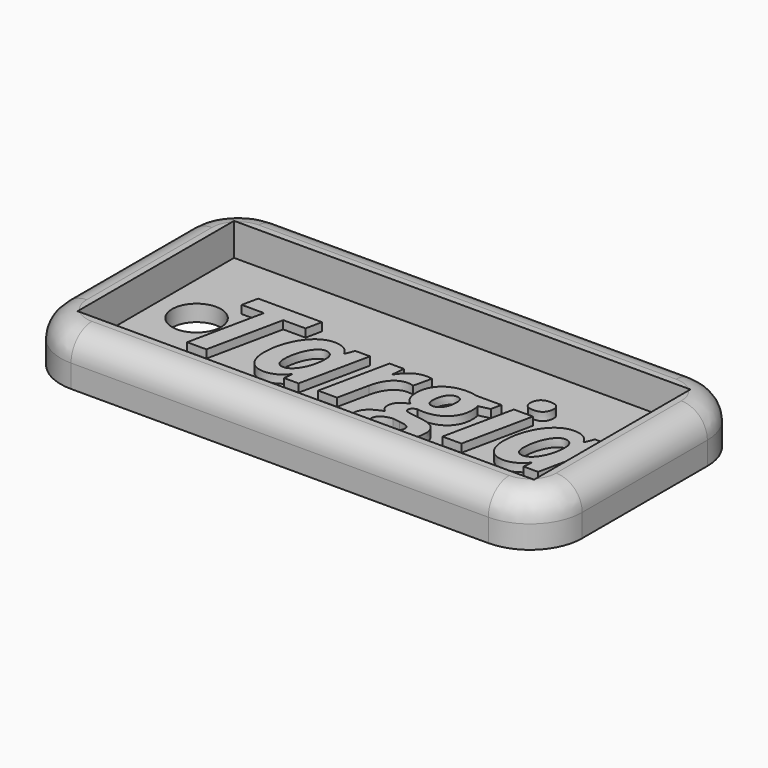
from build123d import *

# Parameters (mm, degrees)
F0_W         = 44.45
F0_H         = 19.05
F0_R         = 2.38125
F1_DEPTH     = 1.5875
F0_W_2       = 50.8
F0_H_2       = 25.4
F2_DEPTH     = 4.7625
F3_R         = 5.08
F4_T1_DEPTH  = 40.64
F4_T3_DEPTH  = 15.24
F4_T6_ANGLE  = 90
F4_T8_ANGLE  = 90
F4_T10_ANGLE = 90
F4_T12_ANGLE = 90
F5_TEXT_SIZE = 12.5911391098
F6_DEPTH     = 0.79375


# Not quite as in the source:
# - a fillet or chamfer that OpenCascade refuses, or shapes differently, is made with other operations: its cross-section is extruded or revolved along the edge and cut away or added
# - Text() gives the source's letters only with a copy of the font that has no kerning and outlines rounded to 1/6400 em; it was checked with that copy


with BuildPart() as f1:
    # F0 (on Top) → F1 (new body)
    with BuildSketch(Plane.XY):
        with Locations((25.4, 12.7)):
            Rectangle(F0_W, F0_H)
        with Locations((7.14375, 12.7)):
            Circle(F0_R, mode=Mode.SUBTRACT)
    extrude(amount=F1_DEPTH)

    # F0 (on Top) → F2 (join)
    with BuildSketch(Plane.XY):
        with Locations((25.4, 12.7)):
            Rectangle(F0_W_2, F0_H_2)
        with Locations((25.4, 12.7)):
            Rectangle(F0_W, F0_H, mode=Mode.SUBTRACT)
    extrude(amount=F2_DEPTH)

    # F3
    f3_edges = [f1.edges().sort_by_distance(p)[0] for p in [
        (50.8, 0, 2.38125),
        (0, 0, 2.38125),
        (50.8, 25.4, 2.38125),
        (0, 25.4, 2.38125),
    ]]
    fillet(f3_edges, radius=F3_R)

    # F4: fillet of radius 2.54 on 8 edges, made by hand

    # F4_s2 → F4_t1 (cut)
    with BuildSketch(Plane.YZ.offset(5.08)):
        with BuildLine():
            ThreePointArc((0, 2.2225), (0.7439487758, 4.0185512242), (2.54, 4.7625))
            Line((2.54, 4.7625), (0, 4.7625))
            Line((0, 4.7625), (0, 2.2225))
        make_face()
        with BuildLine():
            ThreePointArc((25.4, 2.2225), (24.6560512242, 4.0185512242), (22.86, 4.7625))
            Line((22.86, 4.7625), (25.4, 4.7625))
            Line((25.4, 4.7625), (25.4, 2.2225))
        make_face()
    extrude(amount=F4_T1_DEPTH, mode=Mode.SUBTRACT)

    # F4_s4 → F4_t3 (cut)
    with BuildSketch(Plane.XZ.offset(-20.32)):
        with BuildLine():
            ThreePointArc((0, 2.2225), (0.7439487758, 4.0185512242), (2.54, 4.7625))
            Line((2.54, 4.7625), (0, 4.7625))
            Line((0, 4.7625), (0, 2.2225))
        make_face()
        with BuildLine():
            ThreePointArc((50.8, 2.2225), (50.0560512242, 4.0185512242), (48.26, 4.7625))
            Line((48.26, 4.7625), (50.8, 4.7625))
            Line((50.8, 4.7625), (50.8, 2.2225))
        make_face()
    extrude(amount=F4_T3_DEPTH, mode=Mode.SUBTRACT)

    # F4_s5 → F4_t6 (revolve, cut)
    with BuildSketch(Plane.XZ.offset(-20.32)):
        with BuildLine():
            ThreePointArc((0, 2.2225), (0.7439487758, 4.0185512242), (2.54, 4.7625))
            Line((2.54, 4.7625), (0, 4.7625))
            Line((0, 4.7625), (0, 2.2225))
        make_face()
    revolve(axis=Axis((5.08, 20.32, 4.7625), (0, 0, -1)), revolution_arc=F4_T6_ANGLE, mode=Mode.SUBTRACT)

    # F4_s7 → F4_t8 (revolve, cut)
    with BuildSketch(Plane.XZ.offset(-5.08)):
        with BuildLine():
            ThreePointArc((0, 2.2225), (0.7439487758, 4.0185512242), (2.54, 4.7625))
            Line((2.54, 4.7625), (0, 4.7625))
            Line((0, 4.7625), (0, 2.2225))
        make_face()
    revolve(axis=Axis((5.08, 5.08, 4.7625), (0, 0, 1)), revolution_arc=F4_T8_ANGLE, mode=Mode.SUBTRACT)

    # F4_s9 → F4_t10 (revolve, cut)
    with BuildSketch(Plane.XZ.offset(-20.32)):
        with BuildLine():
            ThreePointArc((50.8, 2.2225), (50.0560512242, 4.0185512242), (48.26, 4.7625))
            Line((48.26, 4.7625), (50.8, 4.7625))
            Line((50.8, 4.7625), (50.8, 2.2225))
        make_face()
    revolve(axis=Axis((45.72, 20.32, 4.7625), (0, 0, 1)), revolution_arc=F4_T10_ANGLE, mode=Mode.SUBTRACT)

    # F4_s11 → F4_t12 (revolve, cut)
    with BuildSketch(Plane.YZ.offset(45.72)):
        with BuildLine():
            ThreePointArc((0, 2.2225), (0.7439487758, 4.0185512242), (2.54, 4.7625))
            Line((2.54, 4.7625), (0, 4.7625))
            Line((0, 4.7625), (0, 2.2225))
        make_face()
    revolve(axis=Axis((45.72, 5.08, 4.7625), (0, 0, 1)), revolution_arc=F4_T12_ANGLE, mode=Mode.SUBTRACT)

    # F5 (on face) → F6 (join)
    with BuildSketch(Plane.XY.offset(1.5875)):
        with Locations((8.3821003724, 7.9563454469)):
            Text('Targia', F5_TEXT_SIZE, font='Open Sans', font_style=FontStyle.BOLDITALIC, text_align=(TextAlign.LEFT, TextAlign.BOTTOM))
    extrude(amount=F6_DEPTH)


solid = f1.part
